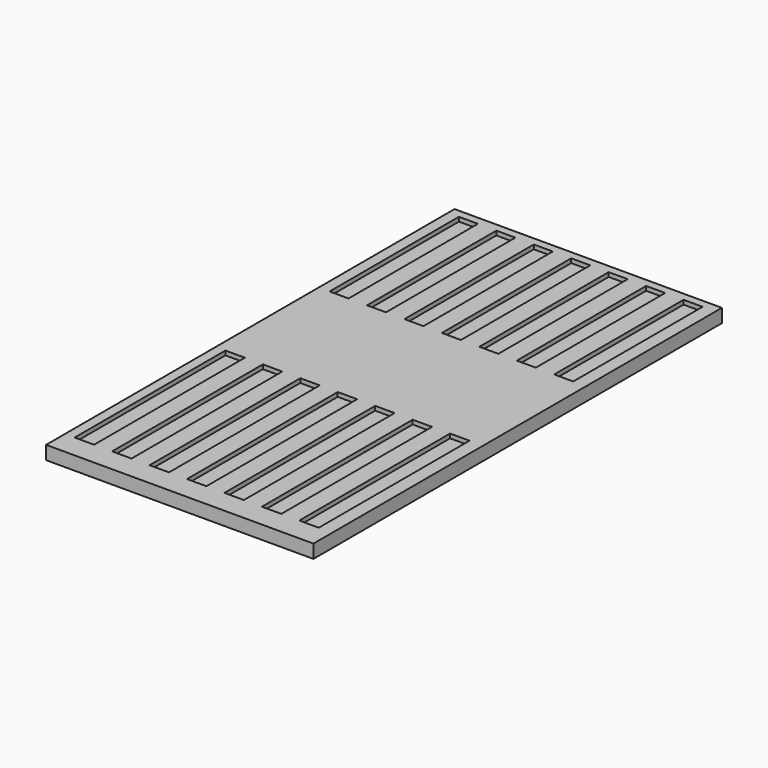
from build123d import *

# Parameters (mm, degrees)
F0_W     = 62.8318530718
F0_H     = 120
F1_DEPTH = 3.175
F2_W     = 4.4705853476
F2_H     = 38
F3_W     = 4.4705853476
F3_H     = 38
F3_W_2   = 4.565641284
F3_H_2   = 44.2867465317
F4_DEPTH = 1


# Not quite as in the source:
# - a length typed as a fraction of an inch, garbled in the dataset ("3 / 203.2 mm" for 3/8 in), is restored


with BuildPart() as f1:
    # F0 (on Top) → F1 (new body)
    with BuildSketch(Plane.XY):
        with Locations((-17.3296490684, 32.2412615943)):
            Rectangle(F0_W, F0_H)
    extrude(amount=F1_DEPTH)

    # F2 (on face) + F3 (on face) → F4 (cut)
    with BuildSketch(Plane.XY.offset(3.175)):
        with Locations((-26.3693033695, 71.3383685797)):
            Rectangle(F2_W, F2_H)
        with Locations((-43.9693033695, 71.3383685797)):
            Rectangle(F2_W, F2_H)
        with Locations((-35.1693033695, 71.3383685797)):
            Rectangle(F2_W, F2_H)
        with Locations((-8.7693033695, 71.3383685797)):
            Rectangle(F2_W, F2_H)
        with Locations((0.0306966305, 71.3383685797)):
            Rectangle(F2_W, F2_H)
        with Locations((8.8306966305, 71.3383685797)):
            Rectangle(F2_W, F2_H)
    with BuildSketch(Plane.XY.offset(3.175)):
        with Locations((-17.5693033695, 71.3383685797)):
            Rectangle(F3_W, F3_H)
        with Locations((-0.1788695753, -0.0753514469)):
            Rectangle(F3_W_2, F3_H_2)
        with Locations((-8.9788695753, -0.0753514469)):
            Rectangle(F3_W_2, F3_H_2)
        with Locations((-17.7788695753, -0.0753514469)):
            Rectangle(F3_W_2, F3_H_2)
        with Locations((-26.5788695753, -0.0753514469)):
            Rectangle(F3_W_2, F3_H_2)
        with Locations((-35.3788695753, -0.0753514469)):
            Rectangle(F3_W_2, F3_H_2)
        with Locations((-44.1788695753, -0.0753514469)):
            Rectangle(F3_W_2, F3_H_2)
        with Locations((8.6211304247, -0.0753514469)):
            Rectangle(F3_W_2, F3_H_2)
    extrude(amount=-F4_DEPTH, mode=Mode.SUBTRACT)


solid = f1.part
